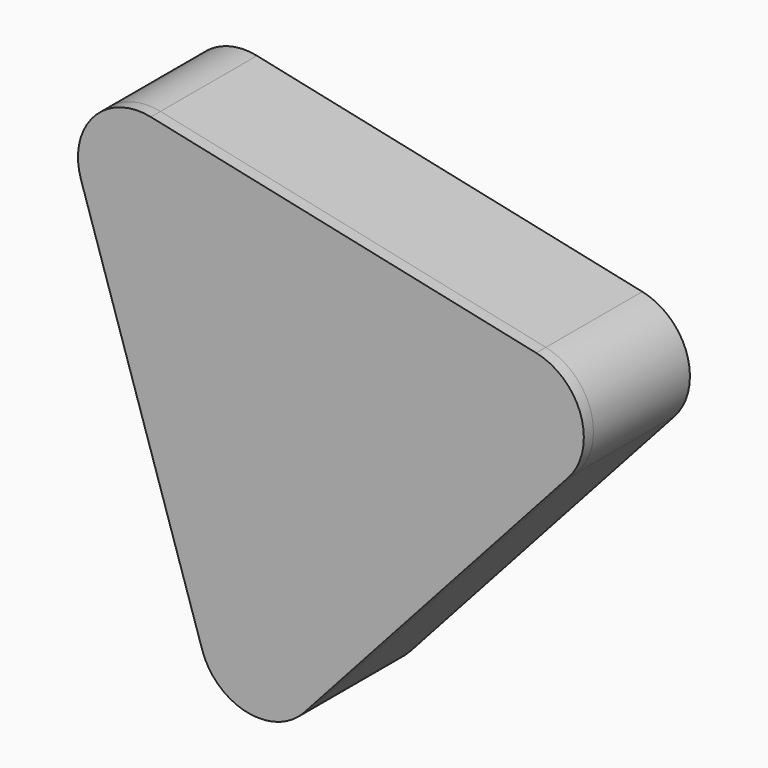
from build123d import *

# Parameters (mm, degrees)
F0_DEPTH = 25.4
F1_R     = 12.7
F2_T     = -2.54
F4_DEPTH = 12.7
F7_DEPTH = 10.16
F9_DEPTH = 2.54


# Not quite as in the source:
# - a feature of the source that left no trace in its solid (it failed there, or was rolled back) is left out


with BuildPart() as f0:
    # F6 (on Front) → F0 (new body)
    with BuildSketch(Plane.XZ):
        Polygon((-15.3317583938, -71.7026534927), (69.7621986403, 22.5736344926), (-54.4304402465, 49.129019), align=None)
    extrude(amount=F0_DEPTH)

    # F1
    f1_edges = [f0.edges().sort_by_distance(p)[0] for p in [
        (69.762199, -12.7, 22.573634),
        (-15.331758, -12.7, -71.702653),
        (-54.43044, -12.7, 49.129019),
    ]]
    fillet(f1_edges, radius=F1_R)

    # F2
    f2_openings = [f0.faces().sort_by_distance(p)[0] for p in [
        (0, -25.4, 0),
    ]]
    offset(amount=F2_T, openings=f2_openings)

    # F3 (on face) → F4 (join)
    with BuildSketch(Plane.XZ.offset(2.54)):
        with BuildLine():
            ThreePointArc((-19.6872152917, -49.9920202635), (-12.1451122529, -56.7995368262), (-2.4785784535, -53.671642278))
            Line((-2.4785784535, -53.671642278), (53.1379671806, 7.9463815593))
            ThreePointArc((53.1379671806, 7.9463815593), (55.2623979412, 17.8817926703), (47.7202949023, 24.689309233))
            Line((47.7202949023, 24.689309233), (-33.4507518888, 42.0456387041))
            ThreePointArc((-33.4507518888, 42.0456387041), (-43.1172856883, 38.9177441559), (-45.2417164489, 28.982333045))
            Line((-45.2417164489, 28.982333045), (-19.6872152917, -49.9920202635))
        make_face()
        with BuildLine():
            Line((-17.2705818419, -49.2100466265), (-42.825082999, 29.7643066821))
            ThreePointArc((-42.825082999, 29.7643066821), (-41.2317599286, 37.2158650153), (-33.981859579, 39.5617859264))
            Line((-33.981859579, 39.5617859264), (47.1891872122, 22.2054564553))
            ThreePointArc((47.1891872122, 22.2054564553), (52.8457644913, 17.0998190332), (51.2524414209, 9.6482607))
            Line((51.2524414209, 9.6482607), (-4.3641042132, -51.9697631373))
            ThreePointArc((-4.3641042132, -51.9697631373), (-11.6140045628, -54.3156840485), (-17.2705818419, -49.2100466265))
        make_face(mode=Mode.SUBTRACT)
    extrude(amount=F4_DEPTH)


with BuildPart() as f7:
    # F7 (new): a face of the model
    f7_faces = [f0.part.faces().sort_by_distance(p)[0] for p in [
        (-11.8482246963, -15.24, -55.4110708034),
    ]]
    extrude(f7_faces, amount=F7_DEPTH)

    # F8 (on face) → F9 (join)
    with BuildSketch(Plane.XZ.offset(25.4)):
        with BuildLine():
            ThreePointArc((55.0234929403, 6.2445024187), (57.679031391, 18.6637663073), (48.2514025925, 27.1731620108))
            Line((48.2514025925, 27.1731620108), (-32.9196441987, 44.5294914819))
            ThreePointArc((-32.9196441987, 44.5294914819), (-45.002811448, 40.6196232966), (-47.6583498987, 28.200359408))
            Line((-47.6583498987, 28.200359408), (-22.1038487416, -50.7739939006))
            ThreePointArc((-22.1038487416, -50.7739939006), (-12.6762199431, -59.283389604), (-0.5930526938, -55.3735214187))
            Line((-0.5930526938, -55.3735214187), (55.0234929403, 6.2445024187))
        make_face()
    extrude(amount=F9_DEPTH)


solid = Compound([f0.part, f7.part])
